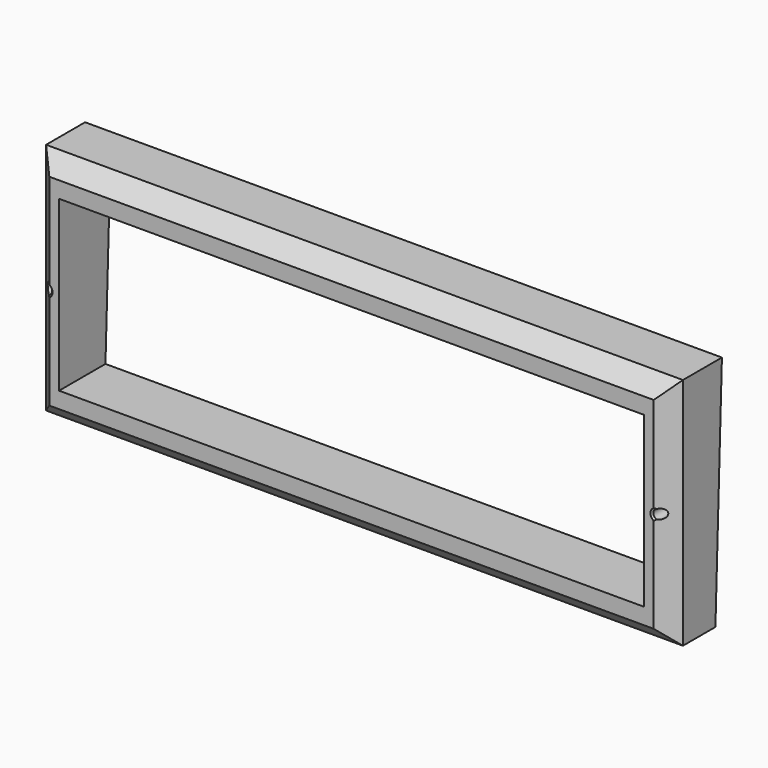
from build123d import *

# Parameters (mm, degrees)
F0_W           = 196
F0_H           = 72
F0_W_2         = 180
F0_H_2         = 52
F1_DEPTH       = 20
F3_DEPTH       = 228.8
F5_D           = 3
F5_DEPTH       = 25
F5_CSINK_D     = 4
F5_CSINK_ANGLE = 90
F5_TIP         = 0.9012909285
F6_T1_DEPTH    = 221.7168298797
F6_T3_DEPTH    = 97.7168298797


# Not quite as in the source:
# - a fillet or chamfer that OpenCascade refuses, or shapes differently, is made with other operations: its cross-section is extruded or revolved along the edge and cut away or added


with BuildPart() as f1:
    # F0 (on Front) → F1 (new body)
    with BuildSketch(Plane.XZ):
        with Locations((1.4274816513, 6.9819294512)):
            Rectangle(F0_W, F0_H)
        with Locations((1.4274816513, 6.9819294512)):
            Rectangle(F0_W_2, F0_H_2, mode=Mode.SUBTRACT)
    extrude(amount=F1_DEPTH)

    # F2 (on face) → F3 (cut)
    with BuildSketch(Plane(origin=(-96.5725183487, 0, 0), x_dir=(0, -1, 0), z_dir=(-1, 0, 0))):
        Polygon((2.5, -29.0180705488), (0, 42.9819294512), (0, -29.0180705488), align=None)
    extrude(amount=-F3_DEPTH, mode=Mode.SUBTRACT)

    # F5
    with Locations(Plane.XZ.offset(20)):
        with Locations((-92.5725183487, 6.9819294512), (95.4274816513, 6.9819294512)):
            CounterSinkHole(F5_D / 2, F5_CSINK_D / 2, depth=F5_DEPTH, counter_sink_angle=F5_CSINK_ANGLE)
            with Locations((0, 0, -(F5_DEPTH + F5_TIP / 2))):  # 118° drill point
                Cone(0, F5_D / 2, F5_TIP, mode=Mode.SUBTRACT)

    # F6: chamfer of 5 on 4 edges, made by hand

    # F6_s2 → F6_t1 (cut)
    with BuildSketch(Plane.YZ.offset(-109.4309332885)):
        Polygon((-15, 42.9819294512), (-20, 37.9819294512), (-20, 42.9819294512), align=None)
        Polygon((-20, -24.0180705488), (-15, -29.0180705488), (-20, -29.0180705488), align=None)
    extrude(amount=F6_T1_DEPTH, mode=Mode.SUBTRACT)

    # F6_s4 → F6_t3 (cut)
    with BuildSketch(Plane.XY.offset(-41.8764854886)):
        Polygon((-91.5725183487, -20), (-96.5725183487, -15), (-96.5725183487, -20), align=None)
        Polygon((99.4274816513, -15), (94.4274816513, -20), (99.4274816513, -20), align=None)
    extrude(amount=F6_T3_DEPTH, mode=Mode.SUBTRACT)


solid = f1.part
